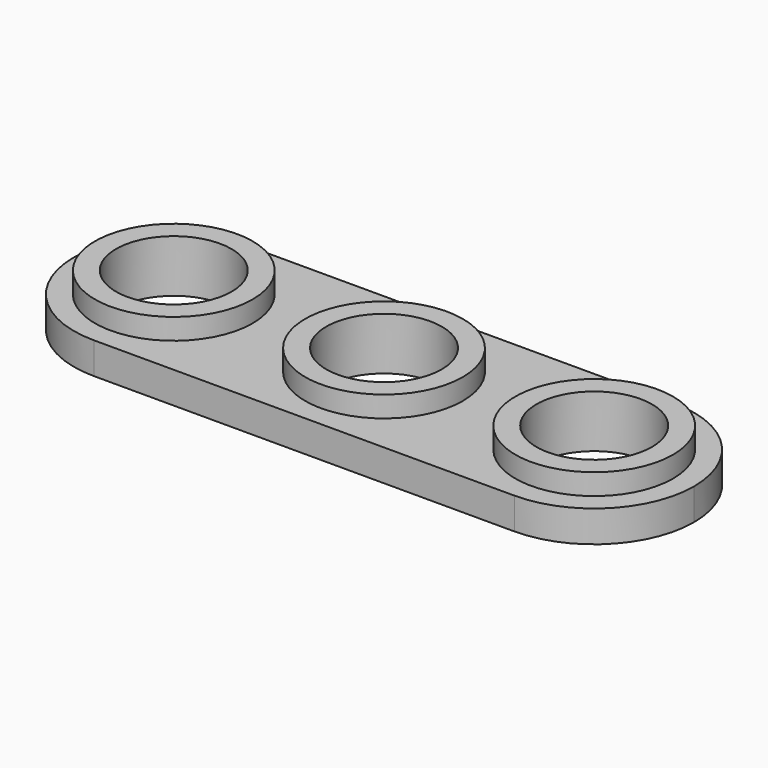
from build123d import *

# Parameters (mm, degrees)
F2_R     = 7.5
F2_R_2   = 5.5
F3_DEPTH = 3
F4_DEPTH = 5


# Not quite as in the source:
# - a feature names something its author has since deleted; it is built from what else it names


with BuildPart() as f3:
    # F2 (on Top) → F3 (new body)
    with BuildSketch(Plane.XY):
        with BuildLine():
            Line((40, 9.5), (0, 9.5))
            ThreePointArc((0, 9.5), (-6.7175144213, 6.7175144213), (-9.5, 0))
            ThreePointArc((-9.5, 0), (-6.7175144213, -6.7175144213), (0, -9.5))
            Line((0, -9.5), (40, -9.5))
            ThreePointArc((40, -9.5), (46.7175144213, -6.7175144213), (49.5, 0))
            ThreePointArc((49.5, 0), (46.7175144213, 6.7175144213), (40, 9.5))
        make_face()
        Circle(F2_R, mode=Mode.SUBTRACT)
        with Locations((20, 0)):
            Circle(F2_R, mode=Mode.SUBTRACT)
        with Locations((40, 0)):
            Circle(F2_R, mode=Mode.SUBTRACT)
        Circle(F2_R)
        Circle(F2_R_2, mode=Mode.SUBTRACT)
        with Locations((20, 0)):
            Circle(F2_R)
        with Locations((20, 0)):
            Circle(F2_R_2, mode=Mode.SUBTRACT)
        with Locations((40, 0)):
            Circle(F2_R)
        with Locations((40, 0)):
            Circle(F2_R_2, mode=Mode.SUBTRACT)
    extrude(amount=F3_DEPTH)

    # F2 (on Top) → F4 (join)
    with BuildSketch(Plane.XY):
        Circle(F2_R)
        Circle(F2_R_2, mode=Mode.SUBTRACT)
        with Locations((20, 0)):
            Circle(F2_R)
        with Locations((20, 0)):
            Circle(F2_R_2, mode=Mode.SUBTRACT)
        with Locations((40, 0)):
            Circle(F2_R)
        with Locations((40, 0)):
            Circle(F2_R_2, mode=Mode.SUBTRACT)
    extrude(amount=F4_DEPTH)


solid = f3.part
